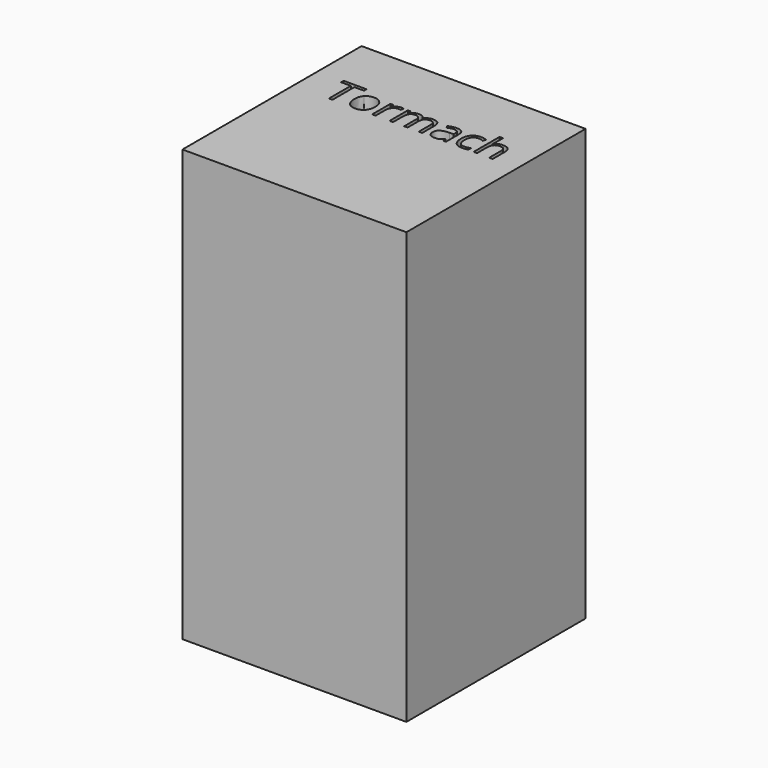
from build123d import *

# Parameters (mm, degrees)
F0_W     = 1016
F0_H     = 1016
F1_DEPTH = 1955.8


with BuildPart() as f1:
    # F0 (on Top) → F1 (new body)
    with BuildSketch(Plane.XY):
        with Locations((52.5003295943, -83.767197299)):
            Rectangle(F0_W, F0_H)
        Polygon((-278.7042081327, 162.2862787117), (-278.7042081327, 37.9848740995), (-294.8145439514, 37.9848740995), (-294.8145439514, 162.2862787117), (-338.7159675476, 162.2862787117), (-338.7159675476, 176.6065772172), (-234.8027845364, 176.6065772172), (-234.8027845364, 162.2862787117), align=None, mode=Mode.SUBTRACT)
        with BuildLine():
            add(Edge.make_bspline(
                [(-139.4605428977, 129.2919468797), (-126.6117157429, 114.7744408736), (-126.6117157429, 90.0476542593)],
                knots=[0, 0, 0, 1, 1, 1], degree=2))
            add(Edge.make_bspline(
                [(-126.6117157429, 90.0476542593), (-126.6117157429, 64.6230564889), (-139.3998636668, 50.3482674067)],
                knots=[0, 0, 0, 1, 1, 1], degree=2))
            add(Edge.make_bspline(
                [(-139.3998636668, 50.3482674067), (-152.1880115906, 36.0734783244), (-174.760685506, 36.0734783244)],
                knots=[0, 0, 0, 1, 1, 1], degree=2))
            add(Edge.make_bspline(
                [(-174.760685506, 36.0734783244), (-188.7169086258, 36.0734783244), (-199.5178117359, 42.6268352676)],
                knots=[0, 0, 0, 1, 1, 1], degree=2))
            add(Edge.make_bspline(
                [(-199.5178117359, 42.6268352676), (-210.3187148459, 49.1801922108), (-216.2046002486, 61.4070572483)],
                knots=[0, 0, 0, 1, 1, 1], degree=2))
            add(Edge.make_bspline(
                [(-216.2046002486, 61.4070572483), (-222.0904856513, 73.6339222858), (-222.0904856513, 90.0476542593)],
                knots=[0, 0, 0, 1, 1, 1], degree=2))
            add(Edge.make_bspline(
                [(-222.0904856513, 90.0476542593), (-222.0904856513, 115.4419124141), (-209.3781867661, 129.6256826499)],
                knots=[0, 0, 0, 1, 1, 1], degree=2))
            add(Edge.make_bspline(
                [(-209.3781867661, 129.6256826499), (-196.665887881, 143.8094528858), (-174.0932139655, 143.8094528858)],
                knots=[0, 0, 0, 1, 1, 1], degree=2))
            add(Edge.make_bspline(
                [(-174.0932139655, 143.8094528858), (-152.3093700525, 143.8094528858), (-139.4605428977, 129.2919468797)],
                knots=[0, 0, 0, 1, 1, 1], degree=2))
        make_face(mode=Mode.SUBTRACT)
        with BuildLine():
            add(Edge.make_bspline(
                [(-69.5125594139, 138.3028126766), (-61.3512028503, 143.8094528858), (-51.5818466665, 143.8094528858)],
                knots=[0, 0, 0, 1, 1, 1], degree=2))
            add(Edge.make_bspline(
                [(-51.5818466665, 143.8094528858), (-44.6644143376, 143.8094528858), (-39.1729439361, 142.6565474976)],
                knots=[0, 0, 0, 1, 1, 1], degree=2))
            Line((-39.1729439361, 142.6565474976), (-41.3573962505, 128.0631924528))
            add(Edge.make_bspline(
                [(-41.3573962505, 128.0631924528), (-47.7893947318, 129.4891543803), (-52.7347520547, 129.4891543803)],
                knots=[0, 0, 0, 1, 1, 1], degree=2))
            add(Edge.make_bspline(
                [(-52.7347520547, 129.4891543803), (-65.3560320934, 129.4891543803), (-74.3062186593, 119.2495341566)],
                knots=[0, 0, 0, 1, 1, 1], degree=2))
            add(Edge.make_bspline(
                [(-74.3062186593, 119.2495341566), (-83.2564052253, 109.0099139328), (-83.2564052253, 93.7490873475)],
                knots=[0, 0, 0, 1, 1, 1], degree=2))
            Line((-83.2564052253, 93.7490873475), (-83.2564052253, 37.9848740995))
            Line((-83.2564052253, 37.9848740995), (-99.0026656582, 37.9848740995))
            Line((-99.0026656582, 37.9848740995), (-99.0026656582, 141.8980571107))
            Line((-99.0026656582, 141.8980571107), (-86.0173102337, 141.8980571107))
            Line((-86.0173102337, 141.8980571107), (-84.1969333051, 122.6627408978))
            Line((-84.1969333051, 122.6627408978), (-83.4384429181, 122.6627408978))
            add(Edge.make_bspline(
                [(-83.4384429181, 122.6627408978), (-77.6739159774, 132.7961724674), (-69.5125594139, 138.3028126766)],
                knots=[0, 0, 0, 1, 1, 1], degree=2))
        make_face(mode=Mode.SUBTRACT)
        with BuildLine():
            Line((128.4534315782, 37.9848740995), (112.7375107608, 37.9848740995))
            Line((112.7375107608, 37.9848740995), (112.7375107608, 105.5815373838))
            add(Edge.make_bspline(
                [(112.7375107608, 105.5815373838), (112.7375107608, 118.0207797297), (107.4280780522, 124.2252310949)],
                knots=[0, 0, 0, 1, 1, 1], degree=2))
            add(Edge.make_bspline(
                [(107.4280780522, 124.2252310949), (102.1186453436, 130.4296824601), (90.9233272323, 130.4296824601)],
                knots=[0, 0, 0, 1, 1, 1], degree=2))
            add(Edge.make_bspline(
                [(90.9233272323, 130.4296824601), (76.2389533411, 130.4296824601), (69.215332358, 121.9952693573)],
                knots=[0, 0, 0, 1, 1, 1], degree=2))
            add(Edge.make_bspline(
                [(69.215332358, 121.9952693573), (62.1917113749, 113.5608562545), (62.1917113749, 96.0245585084)],
                knots=[0, 0, 0, 1, 1, 1], degree=2))
            Line((62.1917113749, 96.0245585084), (62.1917113749, 37.9848740995))
            Line((62.1917113749, 37.9848740995), (46.445450942, 37.9848740995))
            Line((46.445450942, 37.9848740995), (46.445450942, 105.5815373838))
            add(Edge.make_bspline(
                [(46.445450942, 105.5815373838), (46.445450942, 118.0207797297), (41.1360182334, 124.2252310949)],
                knots=[0, 0, 0, 1, 1, 1], degree=2))
            add(Edge.make_bspline(
                [(41.1360182334, 124.2252310949), (35.8265855248, 130.4296824601), (24.5402485671, 130.4296824601)],
                knots=[0, 0, 0, 1, 1, 1], degree=2))
            add(Edge.make_bspline(
                [(24.5402485671, 130.4296824601), (9.7648558294, 130.4296824601), (2.8929329237, 121.5705147406)],
                knots=[0, 0, 0, 1, 1, 1], degree=2))
            add(Edge.make_bspline(
                [(2.8929329237, 121.5705147406), (-3.978989982, 112.7113470211), (-3.978989982, 92.5051631129)],
                knots=[0, 0, 0, 1, 1, 1], degree=2))
            Line((-3.978989982, 92.5051631129), (-3.978989982, 37.9848740995))
            Line((-3.978989982, 37.9848740995), (-19.7252504149, 37.9848740995))
            Line((-19.7252504149, 37.9848740995), (-19.7252504149, 141.8980571107))
            Line((-19.7252504149, 141.8980571107), (-6.9219326833, 141.8980571107))
            Line((-6.9219326833, 141.8980571107), (-4.3734049832, 127.6687774516))
            Line((-4.3734049832, 127.6687774516), (-3.6149145963, 127.6687774516))
            add(Edge.make_bspline(
                [(-3.6149145963, 127.6687774516), (0.845008879, 135.253681321), (8.9608560193, 139.5315671034)],
                knots=[0, 0, 0, 1, 1, 1], degree=2))
            add(Edge.make_bspline(
                [(8.9608560193, 139.5315671034), (17.0767031595, 143.8094528858), (27.1191158827, 143.8094528858)],
                knots=[0, 0, 0, 1, 1, 1], degree=2))
            add(Edge.make_bspline(
                [(27.1191158827, 143.8094528858), (51.4818271113, 143.8094528858), (58.9757121343, 126.1517966777)],
                knots=[0, 0, 0, 1, 1, 1], degree=2))
            Line((58.9757121343, 126.1517966777), (59.7342025212, 126.1517966777))
            add(Edge.make_bspline(
                [(59.7342025212, 126.1517966777), (64.3761636893, 134.3131532412), (73.1898219856, 139.0613030635)],
                knots=[0, 0, 0, 1, 1, 1], degree=2))
            add(Edge.make_bspline(
                [(73.1898219856, 139.0613030635), (82.0034802819, 143.8094528858), (93.2898172396, 143.8094528858)],
                knots=[0, 0, 0, 1, 1, 1], degree=2))
            add(Edge.make_bspline(
                [(93.2898172396, 143.8094528858), (110.9171338321, 143.8094528858), (119.6852827052, 134.7530776657)],
                knots=[0, 0, 0, 1, 1, 1], degree=2))
            add(Edge.make_bspline(
                [(119.6852827052, 134.7530776657), (128.4534315782, 125.6967024456), (128.4534315782, 105.7635750767)],
                knots=[0, 0, 0, 1, 1, 1], degree=2))
            Line((128.4534315782, 105.7635750767), (128.4534315782, 37.9848740995))
        make_face(mode=Mode.SUBTRACT)
        with BuildLine():
            Line((236.4624626789, 37.9848740995), (224.78171072, 37.9848740995))
            Line((224.78171072, 37.9848740995), (221.6567303258, 52.7906064526))
            Line((221.6567303258, 52.7906064526), (220.8982399388, 52.7906064526))
            add(Edge.make_bspline(
                [(220.8982399388, 52.7906064526), (213.1312983765, 43.0212502688), (205.4098662375, 39.5473642966)],
                knots=[0, 0, 0, 1, 1, 1], degree=2))
            add(Edge.make_bspline(
                [(205.4098662375, 39.5473642966), (197.6884340984, 36.0734783244), (186.0987009859, 36.0734783244)],
                knots=[0, 0, 0, 1, 1, 1], degree=2))
            add(Edge.make_bspline(
                [(186.0987009859, 36.0734783244), (170.6558367077, 36.0734783244), (161.8876878347, 44.052797195)],
                knots=[0, 0, 0, 1, 1, 1], degree=2))
            add(Edge.make_bspline(
                [(161.8876878347, 44.052797195), (153.1195389616, 52.0321160657), (153.1195389616, 66.7164899569)],
                knots=[0, 0, 0, 1, 1, 1], degree=2))
            add(Edge.make_bspline(
                [(153.1195389616, 66.7164899569), (153.1195389616, 98.1786712073), (203.4529610391, 99.6956519812)],
                knots=[0, 0, 0, 1, 1, 1], degree=2))
            Line((203.4529610391, 99.6956519812), (221.0802776317, 100.2721046752))
            Line((221.0802776317, 100.2721046752), (221.0802776317, 106.734442772))
            add(Edge.make_bspline(
                [(221.0802776317, 106.734442772), (221.0802776317, 118.9613078095), (215.8315241541, 124.7865139812)],
                knots=[0, 0, 0, 1, 1, 1], degree=2))
            add(Edge.make_bspline(
                [(215.8315241541, 124.7865139812), (210.5827706764, 130.611720153), (198.9930375639, 130.611720153)],
                knots=[0, 0, 0, 1, 1, 1], degree=2))
            add(Edge.make_bspline(
                [(198.9930375639, 130.611720153), (186.0076821395, 130.611720153), (169.6242897815, 122.6627408978)],
                knots=[0, 0, 0, 1, 1, 1], degree=2))
            Line((169.6242897815, 122.6627408978), (164.7699513051, 134.7075682424))
            add(Edge.make_bspline(
                [(164.7699513051, 134.7075682424), (172.4458740209, 138.8640955629), (181.5932680875, 141.2305855702)],
                knots=[0, 0, 0, 1, 1, 1], degree=2))
            add(Edge.make_bspline(
                [(181.5932680875, 141.2305855702), (190.740662154, 143.5970755774), (199.9639052592, 143.5970755774)],
                knots=[0, 0, 0, 1, 1, 1], degree=2))
            add(Edge.make_bspline(
                [(199.9639052592, 143.5970755774), (218.5317499316, 143.5970755774), (227.4971063052, 135.3598699752)],
                knots=[0, 0, 0, 1, 1, 1], degree=2))
            add(Edge.make_bspline(
                [(227.4971063052, 135.3598699752), (236.4624626789, 127.122664373), (236.4624626789, 108.9188950864)],
                knots=[0, 0, 0, 1, 1, 1], degree=2))
            Line((236.4624626789, 108.9188950864), (236.4624626789, 37.9848740995))
        make_face(mode=Mode.SUBTRACT)
        with BuildLine():
            add(Edge.make_bspline(
                [(336.6438729863, 41.5042694949), (326.2373848775, 36.0734783244), (310.4001055981, 36.0734783244)],
                knots=[0, 0, 0, 1, 1, 1], degree=2))
            add(Edge.make_bspline(
                [(310.4001055981, 36.0734783244), (287.8274316827, 36.0734783244), (275.4488685678, 49.9690222132)],
                knots=[0, 0, 0, 1, 1, 1], degree=2))
            add(Edge.make_bspline(
                [(275.4488685678, 49.9690222132), (263.0703054529, 63.864566102), (263.0703054529, 89.2891638723)],
                knots=[0, 0, 0, 1, 1, 1], degree=2))
            add(Edge.make_bspline(
                [(263.0703054529, 89.2891638723), (263.0703054529, 115.3508935677), (275.6460760684, 129.5801732267)],
                knots=[0, 0, 0, 1, 1, 1], degree=2))
            add(Edge.make_bspline(
                [(275.6460760684, 129.5801732267), (288.2218466839, 143.8094528858), (311.4316525243, 143.8094528858)],
                knots=[0, 0, 0, 1, 1, 1], degree=2))
            add(Edge.make_bspline(
                [(311.4316525243, 143.8094528858), (318.9255375473, 143.8094528858), (326.4194225703, 142.1862834577)],
                knots=[0, 0, 0, 1, 1, 1], degree=2))
            add(Edge.make_bspline(
                [(326.4194225703, 142.1862834577), (333.9133075933, 140.5631140296), (338.1608537602, 138.3786617153)],
                knots=[0, 0, 0, 1, 1, 1], degree=2))
            Line((338.1608537602, 138.3786617153), (333.3368548992, 125.0292309051))
            add(Edge.make_bspline(
                [(333.3368548992, 125.0292309051), (328.1184410371, 127.122664373), (321.9594990951, 128.4879470695)],
                knots=[0, 0, 0, 1, 1, 1], degree=2))
            add(Edge.make_bspline(
                [(321.9594990951, 128.4879470695), (315.8005571531, 129.853229766), (311.0675771386, 129.853229766)],
                knots=[0, 0, 0, 1, 1, 1], degree=2))
            add(Edge.make_bspline(
                [(311.0675771386, 129.853229766), (279.3930185799, 129.853229766), (279.3930185799, 89.4712015652)],
                knots=[0, 0, 0, 1, 1, 1], degree=2))
            add(Edge.make_bspline(
                [(279.3930185799, 89.4712015652), (279.3930185799, 70.3269041987), (287.1144507189, 60.087283975)],
                knots=[0, 0, 0, 1, 1, 1], degree=2))
            add(Edge.make_bspline(
                [(287.1144507189, 60.087283975), (294.835882858, 49.8476637513), (310.0056905969, 49.8476637513)],
                knots=[0, 0, 0, 1, 1, 1], degree=2))
            add(Edge.make_bspline(
                [(310.0056905969, 49.8476637513), (322.9910460213, 49.8476637513), (336.6438729863, 55.4301529992)],
                knots=[0, 0, 0, 1, 1, 1], degree=2))
            Line((336.6438729863, 55.4301529992), (336.6438729863, 41.5042694949))
        make_face(mode=Mode.SUBTRACT)
        with BuildLine():
            Line((448.1722994824, 37.9848740995), (432.4260390495, 37.9848740995))
            Line((432.4260390495, 37.9848740995), (432.4260390495, 105.2174619981))
            add(Edge.make_bspline(
                [(432.4260390495, 105.2174619981), (432.4260390495, 117.8994212678), (426.646342301, 124.1645518639)],
                knots=[0, 0, 0, 1, 1, 1], degree=2))
            add(Edge.make_bspline(
                [(426.646342301, 124.1645518639), (420.8666455525, 130.4296824601), (408.518422053, 130.4296824601)],
                knots=[0, 0, 0, 1, 1, 1], degree=2))
            add(Edge.make_bspline(
                [(408.518422053, 130.4296824601), (392.1350296951, 130.4296824601), (384.5956352488, 121.5098355096)],
                knots=[0, 0, 0, 1, 1, 1], degree=2))
            add(Edge.make_bspline(
                [(384.5956352488, 121.5098355096), (377.0562408026, 112.5899885592), (377.0562408026, 92.3231254201)],
                knots=[0, 0, 0, 1, 1, 1], degree=2))
            Line((377.0562408026, 92.3231254201), (377.0562408026, 37.9848740995))
            Line((377.0562408026, 37.9848740995), (361.3099803697, 37.9848740995))
            Line((361.3099803697, 37.9848740995), (361.3099803697, 185.5264241676))
            Line((361.3099803697, 185.5264241676), (377.0562408026, 185.5264241676))
            Line((377.0562408026, 185.5264241676), (377.0562408026, 140.8665101844))
            add(Edge.make_bspline(
                [(377.0562408026, 140.8665101844), (377.0562408026, 132.7961724674), (376.2977504157, 127.4867397588)],
                knots=[0, 0, 0, 1, 1, 1], degree=2))
            Line((376.2977504157, 127.4867397588), (377.2382784955, 127.4867397588))
            add(Edge.make_bspline(
                [(377.2382784955, 127.4867397588), (381.8802396636, 134.9806247817), (390.4663508438, 139.2888501796)],
                knots=[0, 0, 0, 1, 1, 1], degree=2))
            add(Edge.make_bspline(
                [(390.4663508438, 139.2888501796), (399.052462024, 143.5970755774), (410.0354028269, 143.5970755774)],
                knots=[0, 0, 0, 1, 1, 1], degree=2))
            add(Edge.make_bspline(
                [(410.0354028269, 143.5970755774), (429.0886813469, 143.5970755774), (438.6304904147, 134.5407003573)],
                knots=[0, 0, 0, 1, 1, 1], degree=2))
            add(Edge.make_bspline(
                [(438.6304904147, 134.5407003573), (448.1722994824, 125.4843251372), (448.1722994824, 105.7635750767)],
                knots=[0, 0, 0, 1, 1, 1], degree=2))
            Line((448.1722994824, 105.7635750767), (448.1722994824, 37.9848740995))
        make_face(mode=Mode.SUBTRACT)
    extrude(amount=F1_DEPTH)


solid = f1.part
